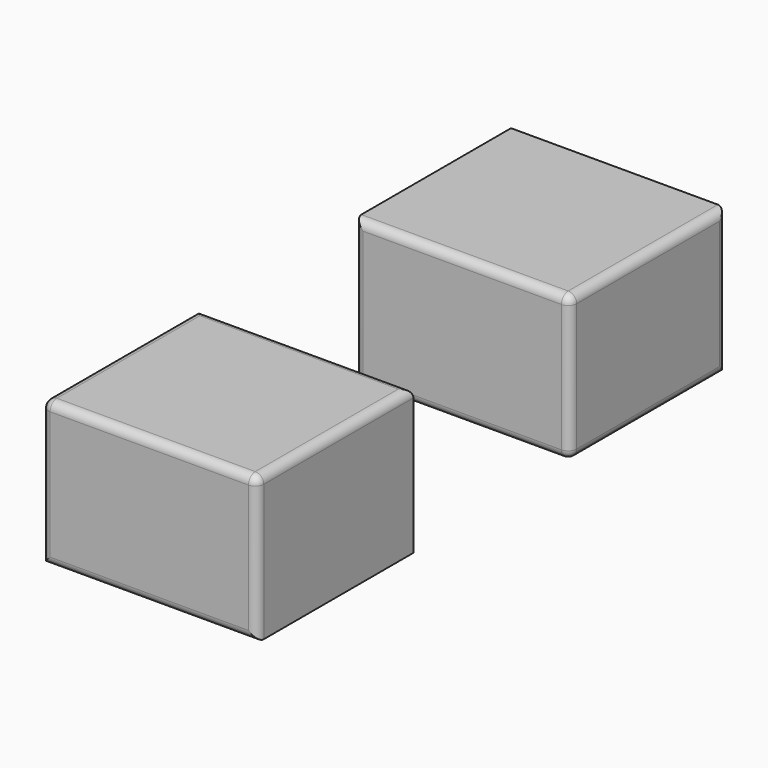
from build123d import *

# Parameters (mm, degrees)
F0_W     = 127.3354738951
F0_H     = 115.6546771526
F1_DEPTH = 85.66379
F4_R     = 5
F4_2_R   = 5


with BuildPart() as f1:
    # F0 (on Top) → F1 (new body)
    with BuildSketch(Plane.XY):
        Rectangle(F0_W, F0_H)
    extrude(amount=F1_DEPTH)


with BuildPart() as f2_1:
    # F2: copy of F1
    add(f1.part.moved(Location((0, 115.6546771526, 0))))


with BuildPart() as f2_1_1:
    # F3: moved
    add(f2_1.part.moved(Location((0, 115.6546771526, 0))))

    # F4
    f4_edges = [f2_1_1.edges().sort_by_distance(p)[0] for p in [
        (63.667737, 173.482016, 42.831895),
        (63.667737, 289.136693, 42.831895),
        (63.667737, 231.309354, 0),
        (63.667737, 231.309354, 85.66379),
        (-63.667737, 173.482016, 42.831895),
        (0, 173.482016, 0),
        (0, 173.482016, 85.66379),
    ]]
    fillet(f4_edges, radius=F4_R)


with BuildPart() as f1_1:
    add(f1.part)

    # F4#2
    f4_2_edges = [f1_1.edges().sort_by_distance(p)[0] for p in [
        (-63.667737, 0, 85.66379),
        (0, -57.827339, 85.66379),
        (63.667737, 0, 85.66379),
        (0, 57.827339, 85.66379),
        (-63.667737, -57.827339, 42.831895),
        (63.667737, -57.827339, 42.831895),
        (0, -57.827339, 0),
    ]]
    fillet(f4_2_edges, radius=F4_2_R)


solid = Compound([f2_1_1.part, f1_1.part])
